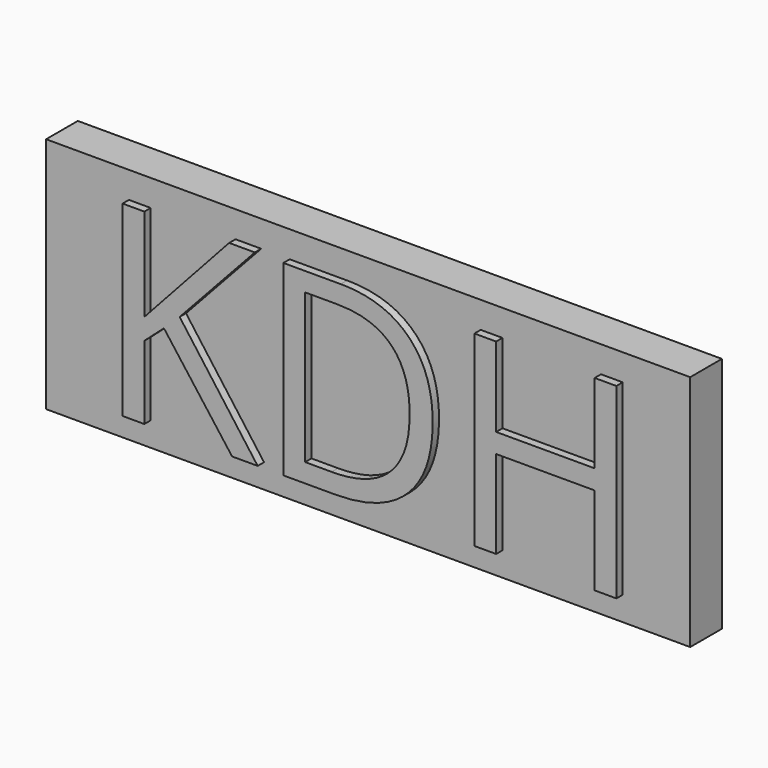
from build123d import *

# Parameters (mm, degrees)
F0_W         = 81.2083035707
F0_H         = 29.9576614052
F1_DEPTH     = 5
F2_TEXT_SIZE = 33.0302434223
F3_DEPTH     = 1


# Not quite as in the source:
# - Text() gives the source's letters only with a copy of the font that has no kerning and outlines rounded to 1/6400 em; it was checked with that copy


with BuildPart() as f1:
    # F0 (on Front) → F1 (new body)
    with BuildSketch(Plane.XZ):
        with Locations((40.6041517854, 14.9788307026)):
            Rectangle(F0_W, F0_H)
    extrude(amount=F1_DEPTH)

    # F2 (on face) → F3 (join)
    with BuildSketch(Plane.XZ.offset(5)):
        with Locations((7.2051989846, 3.0418552924)):
            Text('KDH', F2_TEXT_SIZE, font='Open Sans', text_align=(TextAlign.LEFT, TextAlign.BOTTOM))
    extrude(amount=F3_DEPTH)


solid = f1.part
